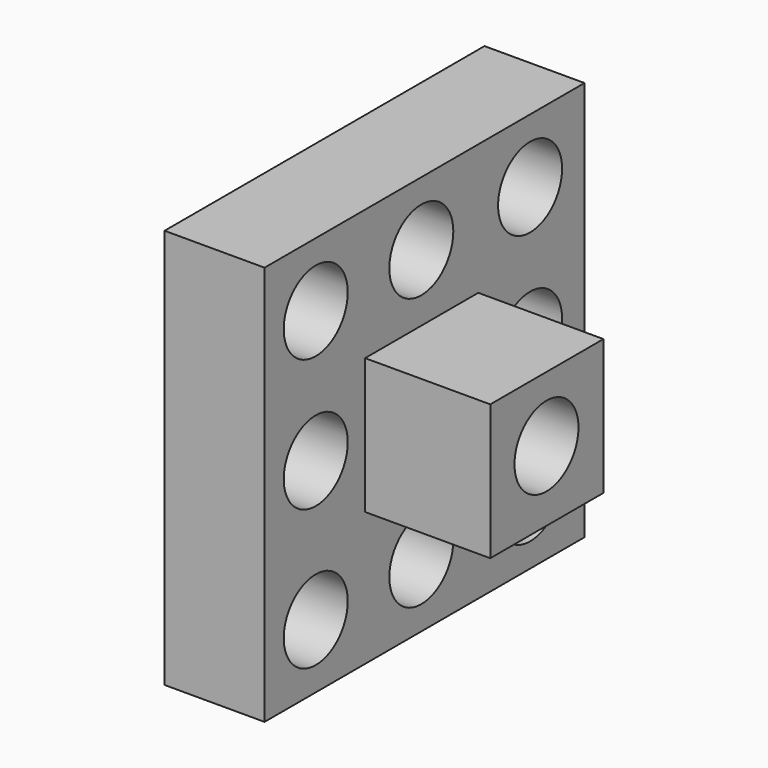
from build123d import *

# Parameters (mm, degrees)
F0_W     = 33
F0_H     = 34
F0_R     = 10
F0_H_2   = 33
F0_W_2   = 34
F1_DEPTH = 25
F2_W     = 35.366706574
F2_H     = 33.8733626366
F2_W_2   = 35.166706574
F2_H_2   = 33.6733626366
F2_R     = 10
F3_DEPTH = 56.3


# Not quite as in the source:
# - a feature names something its author has since deleted; it is built from what else it names


with BuildPart() as f1:
    # F0 (on Right) → F1 (new body)
    with BuildSketch(Plane.YZ):
        with Locations((16.5, 50)):
            Rectangle(F0_W, F0_H)
        with Locations((16, 51)):
            Circle(F0_R, mode=Mode.SUBTRACT)
        with Locations((16.5, 83.5)):
            Rectangle(F0_W, F0_H_2)
        with Locations((16, 84)):
            Circle(F0_R, mode=Mode.SUBTRACT)
        with Locations((50, 83.5)):
            Rectangle(F0_W_2, F0_H_2)
        with Locations((49, 84)):
            Circle(F0_R, mode=Mode.SUBTRACT)
        with Locations((16.5, 16.5)):
            Rectangle(F0_W, F0_H_2)
        with Locations((16, 16)):
            Circle(F0_R, mode=Mode.SUBTRACT)
        with Locations((50, 50)):
            Rectangle(F0_W_2, F0_H)
        with Locations((49, 51)):
            Circle(F0_R, mode=Mode.SUBTRACT)
        with Locations((50, 16.5)):
            Rectangle(F0_W_2, F0_H_2)
        with Locations((49, 16)):
            Circle(F0_R, mode=Mode.SUBTRACT)
        with Locations((83.5, 16.5)):
            Rectangle(F0_W, F0_H_2)
        with Locations((83, 16)):
            Circle(F0_R, mode=Mode.SUBTRACT)
        with Locations((83.5, 50)):
            Rectangle(F0_W, F0_H)
        with Locations((83, 51)):
            Circle(F0_R, mode=Mode.SUBTRACT)
        with Locations((83.5, 83.5)):
            Rectangle(F0_W, F0_H_2)
        with Locations((83, 84)):
            Circle(F0_R, mode=Mode.SUBTRACT)
    extrude(amount=F1_DEPTH)

    # F2 (on Right) → F3 (join)
    with BuildSketch(Plane.YZ):
        with Locations((49.116646713, 50.3734805703)):
            Rectangle(F2_W, F2_H)
        with Locations((49.116646713, 50.3734805703)):
            Rectangle(F2_W_2, F2_H_2, mode=Mode.SUBTRACT)
        with Locations((49.116646713, 50.3734805703)):
            Rectangle(F2_W_2, F2_H_2)
        with Locations((49, 51)):
            Circle(F2_R, mode=Mode.SUBTRACT)
    extrude(amount=F3_DEPTH)


solid = f1.part
